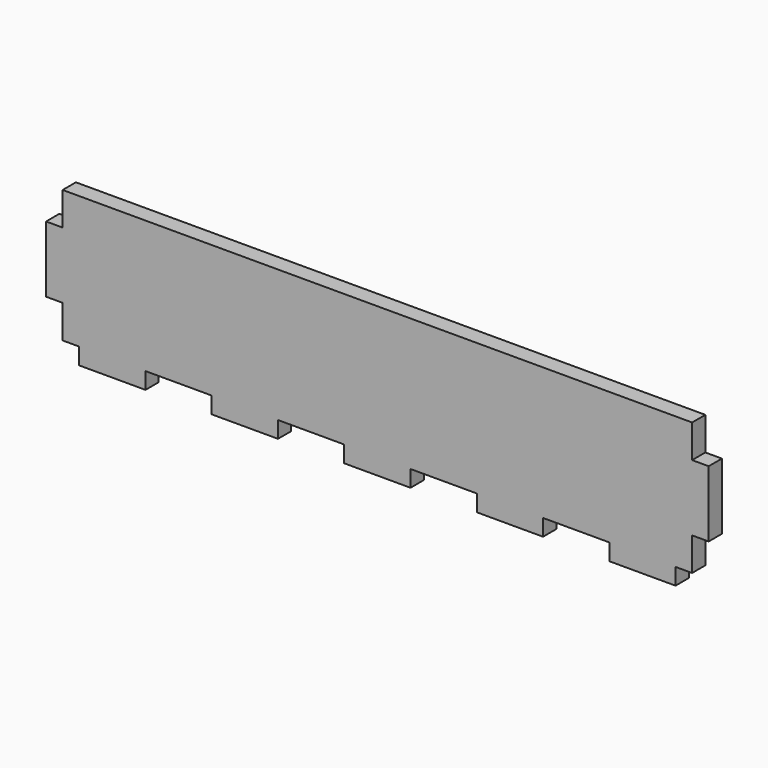
from build123d import *

# Parameters (mm, degrees)
F0_W     = 12.7
F0_H     = 3.175
F0_W_2   = 3.175
F0_H_2   = 12.7
F1_DEPTH = 3.175


# Not quite as in the source:
# - a feature names something its author has since deleted; it is built from what else it names


with BuildPart() as f1:
    # F0 (on Front) → F1 (new body)
    with BuildSketch(Plane.XZ):
        Polygon((15.7950905681, 13.6112950251), (-104.8549094319, 13.6112950251), (-104.8549094319, 7.2612950251), (-104.8549094319, -5.4387049749), (-104.8549094319, -11.7887049749), (-101.6799094319, -11.7887049749), (-88.9799094319, -11.7887049749), (-76.2799094319, -11.7887049749), (-63.5799094319, -11.7887049749), (-50.8799094319, -11.7887049749), (-38.1799094319, -11.7887049749), (-25.4799094319, -11.7887049749), (-12.7799094319, -11.7887049749), (-0.0799094319, -11.7887049749), (12.6200905681, -11.7887049749), (15.7950905681, -11.7887049749), (15.7950905681, -5.4387049749), (15.7950905681, 7.2612950251), align=None)
        with Locations((-44.5299094319, -13.3762049749)):
            Rectangle(F0_W, F0_H)
        with Locations((-19.1299094319, -13.3762049749)):
            Rectangle(F0_W, F0_H)
        with Locations((-95.3299094319, -13.3762049749)):
            Rectangle(F0_W, F0_H)
        with Locations((-69.9299094319, -13.3762049749)):
            Rectangle(F0_W, F0_H)
        with Locations((6.2700905681, -13.3762049749)):
            Rectangle(F0_W, F0_H)
        with Locations((-106.4424094319, 0.9112950251)):
            Rectangle(F0_W_2, F0_H_2)
        with Locations((17.3825905681, 0.9112950251)):
            Rectangle(F0_W_2, F0_H_2)
    extrude(amount=F1_DEPTH)


solid = f1.part
